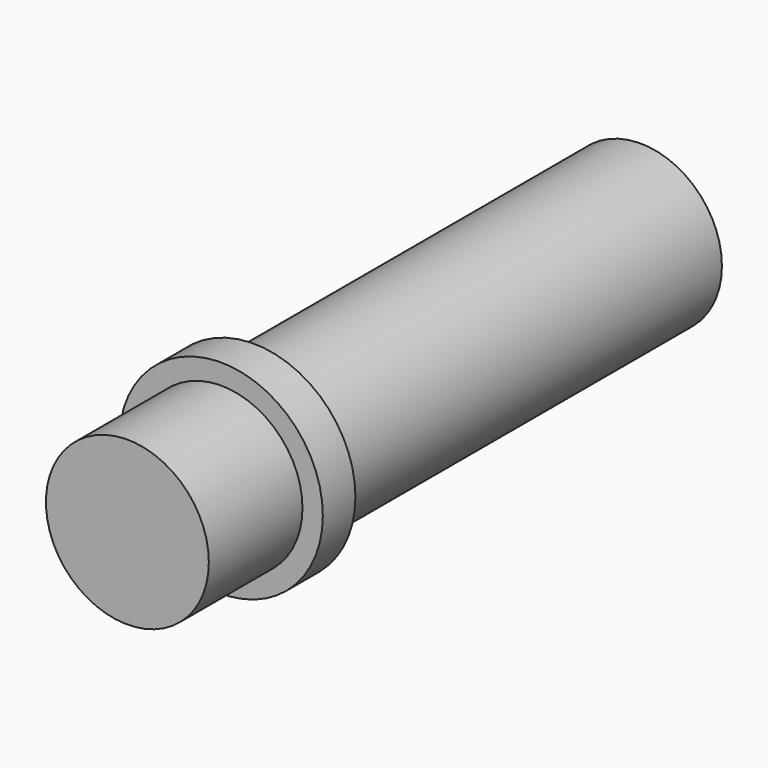
from build123d import *

# Parameters (mm, degrees)
F0_R     = 12.7
F1_DEPTH = 25.4
F2_R     = 15.875
F2_R_2   = 12.7
F3_DEPTH = 6.35
F4_R     = 12.7
F5_DEPTH = 18.2499
F6_DEPTH = 50


# Not quite as in the source:
# - a feature names something its author has since deleted; it is built from what else it names


with BuildPart() as f1:
    # F0 (on Front) → F1 (new body)
    with BuildSketch(Plane.XZ):
        Circle(F0_R)
    extrude(amount=F1_DEPTH)

    # F6 (add): a face of the model
    f6_faces = [f1.faces().sort_by_distance(p)[0] for p in [
        (0, 0, 0),
    ]]
    extrude(f6_faces, amount=F6_DEPTH)


with BuildPart() as f3:
    # F2 (on face) → F3 (new body)
    with BuildSketch(Plane.XZ.offset(25.4)):
        Circle(F2_R)
        Circle(F2_R_2, mode=Mode.SUBTRACT)
        Circle(F2_R_2)
    extrude(amount=F3_DEPTH)

    # F4 (on face) → F5 (join)
    with BuildSketch(Plane.XZ.offset(31.75)):
        Circle(F4_R)
    extrude(amount=F5_DEPTH)


solid = Compound([f1.part, f3.part])
